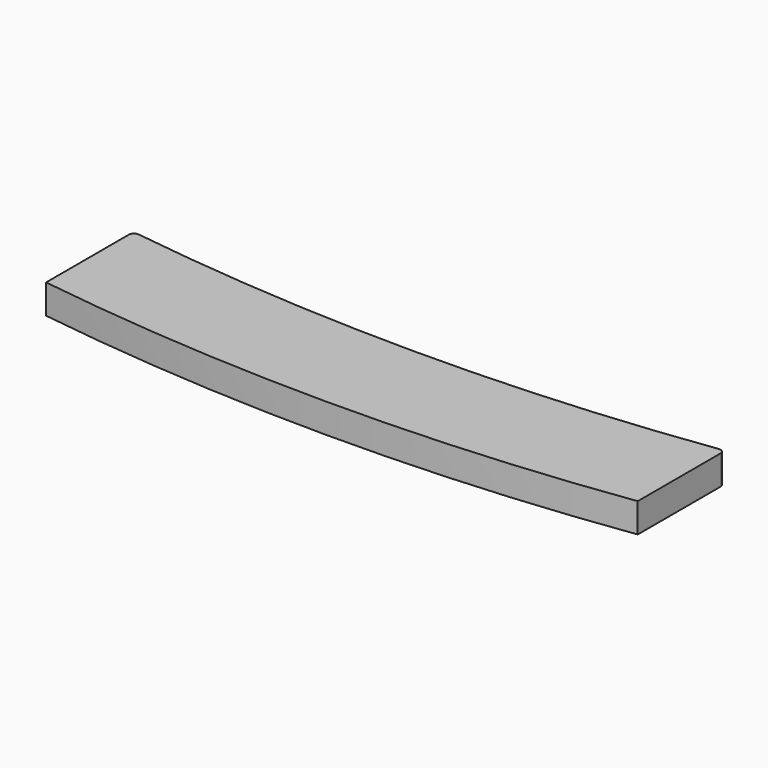
from build123d import *

# Parameters (mm, degrees)
F1_DEPTH = 5.75


# Not quite as in the source:
# - ends of sketch curves that miss each other by under 0.0002 mm in the source are joined


with BuildPart() as f1:
    # F0 (on Top) → F1 (new body)
    with BuildSketch(Plane.XY):
        with BuildLine():
            ThreePointArc((-54.3633709611, 8.0368382821), (-55.1570277624, 7.8000823804), (-55.5, 7.046216))
            Line((-55.5, 7.046216), (-55.5, -13.228097))
            ThreePointArc((-55.5, -13.228097), (2.4981253193, -17.3024292075), (60.5000000667, -13.2818254774))
            Line((60.5000000667, -13.2818254774), (60.5, 6.993434))
            ThreePointArc((60.5, 6.993434), (60.1573766387, 7.7469961772), (59.3642880901, 7.9841823422))
            ThreePointArc((59.3642880901, 7.9841823422), (2.4986576004, 4.1208007581), (-54.3633709611, 8.0368382821))
        make_face()
    extrude(amount=F1_DEPTH)


solid = f1.part
